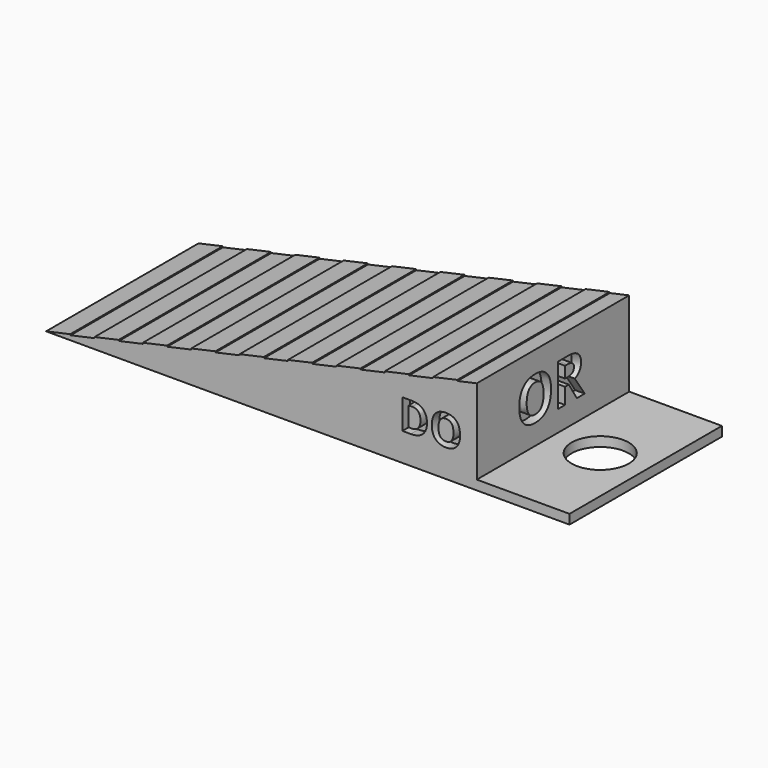
from build123d import *

# Parameters (mm, degrees)
F1_DEPTH      = 25.4
F1_DEPTH_BACK = 25.4
F2_W          = 24.7169253703
F2_H          = 50.8
F3_DEPTH      = 2.54
F5_D          = 15.24
F6_TEXT_SIZE  = 11.4448077511
F7_DEPTH      = 1.27
F8_TEXT_SIZE  = 11.0839778143
F9_DEPTH      = 2.54
F10_TEXT_SIZE = 15.5996686469
F11_DEPTH     = 2.54
F12_TEXT_SIZE = 11.4282903572
F13_DEPTH     = 2.54
F14_W         = 6.604
F14_H         = 50.8
F14_W_2       = 5.3486987998
F15_DEPTH     = 0.254


# Not quite as in the source:
# - Text() gives the source's letters only with a copy of the font that has no kerning and outlines rounded to 1/6400 em; it was checked with that copy


with BuildPart() as f1:
    # F0 (on Front) → F1 (new body, two sides)
    with BuildSketch(Plane.XZ) as f1_sk:
        Polygon((51.5911467373, -15.2608209014), (-63.250169158, -40.6608209014), (51.5911467373, -40.6608209014), align=None)
    extrude(amount=F1_DEPTH)
    extrude(f1_sk.sketch, amount=-F1_DEPTH_BACK)

    # F2 (on face) → F3 (join)
    with BuildSketch(Plane(origin=(0, 0, -40.6608209014), x_dir=(1, 0, 0), z_dir=(0, 0, -1))):
        with Locations((63.9496094225, 0)):
            Rectangle(F2_W, F2_H)
    extrude(amount=-F3_DEPTH)

    # F5 (through all)
    with Locations(Plane.XY.offset(-38.1208209014)):
        with Locations((64.1786307096, 0)):
            Hole(F5_D / 2)

    # F6 (on face) → F7 (cut)
    with BuildSketch(Plane(origin=(0, 0, -40.6608209014), x_dir=(1, 0, 0), z_dir=(0, 0, -1))):
        with Locations((-34.6078742296, 5.9987020213)):
            Text('Do or Stop', F6_TEXT_SIZE, font='Open Sans', font_style=FontStyle.BOLD, text_align=(TextAlign.LEFT, TextAlign.BOTTOM))
        with Locations((-34.6078742296, -9.5662365202)):
            Text('Made by ECH', F6_TEXT_SIZE, font='Open Sans', font_style=FontStyle.BOLD, text_align=(TextAlign.LEFT, TextAlign.BOTTOM))
    extrude(amount=-F7_DEPTH, mode=Mode.SUBTRACT)

    # F8 (on face) → F9 (cut)
    with BuildSketch(Plane.XZ.offset(25.4)):
        with Locations((30.7496581227, -33.1480167806)):
            Text('DO', F8_TEXT_SIZE, font='Open Sans', font_style=FontStyle.BOLD, text_align=(TextAlign.LEFT, TextAlign.BOTTOM))
    extrude(amount=-F9_DEPTH, mode=Mode.SUBTRACT)

    # F10 (on face) → F11 (cut)
    with BuildSketch(Plane.YZ.offset(51.5911467373)):
        with Locations((-12.1624181047, -32.5568709522)):
            Text('OR', F10_TEXT_SIZE, font='Open Sans', font_style=FontStyle.BOLD, text_align=(TextAlign.LEFT, TextAlign.BOTTOM))
    extrude(amount=-F11_DEPTH, mode=Mode.SUBTRACT)

    # F12 (on face) → F13 (cut)
    with BuildSketch(Plane(origin=(0, 25.4, 0), x_dir=(-1, 0, 0), z_dir=(0, 1, 0))):
        with Locations((-49.3963006884, -32.0113711059)):
            Text('STOP', F12_TEXT_SIZE, font='Open Sans', font_style=FontStyle.BOLD, text_align=(TextAlign.LEFT, TextAlign.BOTTOM))
    extrude(amount=-F13_DEPTH, mode=Mode.SUBTRACT)

    # F14 (on face) → F15 (cut)
    with BuildSketch(Plane(origin=(5.6239444679, 0, -25.4276056386), x_dir=(0.9764031559, 0, 0.2159557296), z_dir=(-0.2159557296, 0, 0.9764031559))):
        with Locations((-60.6326020204, 0)):
            Rectangle(F14_W, F14_H)
        with Locations((-47.4246020204, 0)):
            Rectangle(F14_W, F14_H)
        with Locations((-7.8006020204, 0)):
            Rectangle(F14_W, F14_H)
        with Locations((5.4073979796, 0)):
            Rectangle(F14_W, F14_H)
        with Locations((18.6153979796, 0)):
            Rectangle(F14_W, F14_H)
        with Locations((31.8233979796, 0)):
            Rectangle(F14_W, F14_H)
        with Locations((44.4037473795, 0)):
            Rectangle(F14_W_2, F14_H)
        with Locations((-34.2166020204, 0)):
            Rectangle(F14_W, F14_H)
        with Locations((-21.0086020204, 0)):
            Rectangle(F14_W, F14_H)
    extrude(amount=-F15_DEPTH, mode=Mode.SUBTRACT)


solid = f1.part
